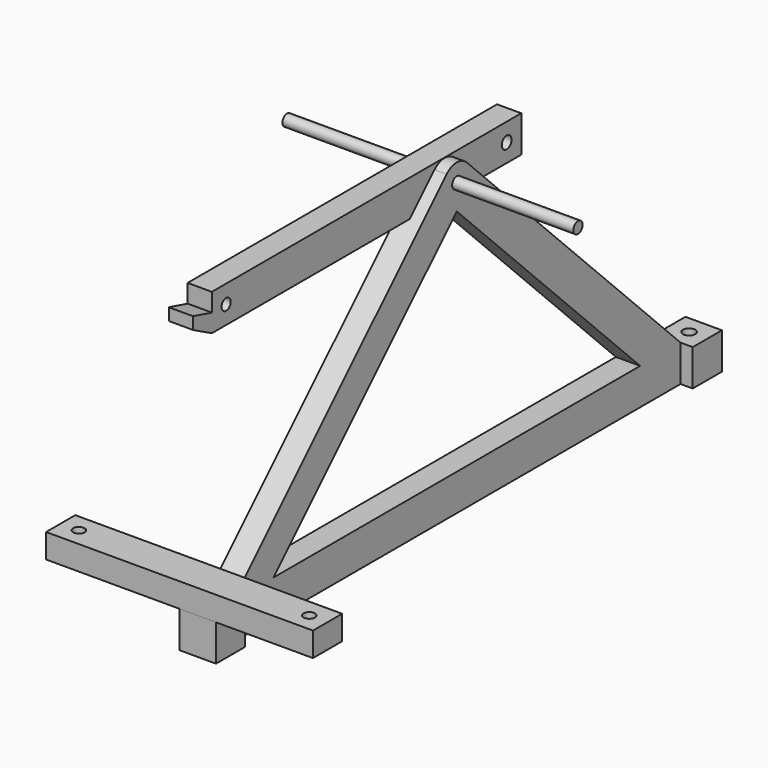
from build123d import *

# Parameters (mm, degrees)
F5_W      = 9.55
F5_H      = 9.55
F7_DEPTH  = 9.55
F5_R      = 1.5
F8_DEPTH  = 6.35
F5_H_2    = 6.35
F9_DEPTH  = 34.95
F10_R     = 1.5
F11_DEPTH = 6.35
F12_R     = 1.6
F13_DEPTH = 9.55
F6_R      = 1.5
F6_R_2    = 1.6
F14_DEPTH = 3.175
F15_DEPTH = 38.1


# Not quite as in the source:
# - a length typed as a fraction of an inch, garbled in the dataset ("3 / 203.2 mm" for 3/8 in), is restored


with BuildPart() as f7:
    # F5 (on Right) → F7 (new body)
    with BuildSketch(Plane.YZ):
        with Locations((-78.0364484041, 4.775)):
            Rectangle(F5_W, F5_H)
    extrude(amount=F7_DEPTH)



with BuildPart() as f7b:
    # F5 (on Right) → F7, piece 2 (new body)
    with BuildSketch(Plane.YZ):
        with Locations((78.0364484041, 4.775)):
            Rectangle(F5_W, F5_H)
    extrude(amount=F7_DEPTH)


with BuildPart() as f7_1:
    add(f7.part)

    add(f7b.part)  # F8 merges F7b
    # F5 (on Right) → F8 (join)
    with BuildSketch(Plane.YZ):
        with BuildLine():
            Line((-3.305724202, 79.505724202), (-73.2614484041, 9.55))
            Line((-73.2614484041, 9.55), (-60.0385515959, 9.55))
            Line((-60.0385515959, 9.55), (0, 69.5885515959))
            Line((0, 69.5885515959), (60.0385515959, 9.55))
            Line((60.0385515959, 9.55), (73.2614484041, 9.55))
            Line((73.2614484041, 9.55), (3.305724202, 79.505724202))
            ThreePointArc((3.305724202, 79.505724202), (0, 80.875), (-3.305724202, 79.505724202))
        make_face()
        with Locations((0, 76.2)):
            Circle(F5_R, mode=Mode.SUBTRACT)
        Polygon((-73.2614484041, 9.55), (-73.2614484041, 0), (73.2614484041, 0), (73.2614484041, 9.55), (60.0385515959, 9.55), (-60.0385515959, 9.55), align=None)
    extrude(amount=F8_DEPTH)

    # F12 (on face) → F13 (cut, through all)
    with BuildSketch(Plane(origin=(0, 0, 0), x_dir=(1, 0, 0), z_dir=(0, 0, -1))):
        with Locations((4.775, 78.0364484041)):
            Circle(F12_R)
        with Locations((4.775, -78.0364484041)):
            Circle(F12_R)
    extrude(amount=-F13_DEPTH, mode=Mode.SUBTRACT)


with BuildPart() as f9:
    # F5 (on Right) → F9 (new body, symmetric)
    with BuildSketch(Plane.YZ):
        with Locations((-78.0364484041, 12.725)):
            Rectangle(F5_W, F5_H_2)
    extrude(amount=F9_DEPTH, both=True)

    # F10 (on face) → F11 (cut, through all)
    with BuildSketch(Plane.XY.offset(15.9)):
        with Locations((30.175, -78.0364484041)):
            Circle(F10_R)
        with Locations((-30.175, -78.0364484041)):
            Circle(F10_R)
    extrude(amount=-F11_DEPTH, mode=Mode.SUBTRACT)


with BuildPart() as f14:
    # F6 (on Right) → F14 (new body, symmetric)
    with BuildSketch(Plane.YZ):
        Polygon((25.095, 80.975), (-76.2, 80.975), (-76.2, 76.2), (-76.2, 71.425), (25.095, 71.425), align=None)
        with Locations((-71.525, 76.2)):
            Circle(F6_R, mode=Mode.SUBTRACT)
        with Locations((0, 76.2)):
            Circle(F6_R_2, mode=Mode.SUBTRACT)
        with Locations((20.32, 76.2)):
            Circle(F6_R_2, mode=Mode.SUBTRACT)
        Polygon((-76.2, 71.425), (-76.2, 76.2), (-82.3336289969, 77.8435009364), (-82.3336289969, 74.6685009364), align=None)
    extrude(amount=F14_DEPTH, both=True)


with BuildPart() as f15:
    # F5 (on Right) → F15 (new body, symmetric)
    with BuildSketch(Plane.YZ):
        with Locations((0, 76.2)):
            Circle(F5_R)
    extrude(amount=F15_DEPTH, both=True)


solid = Compound([f7_1.part, f9.part, f14.part, f15.part])
